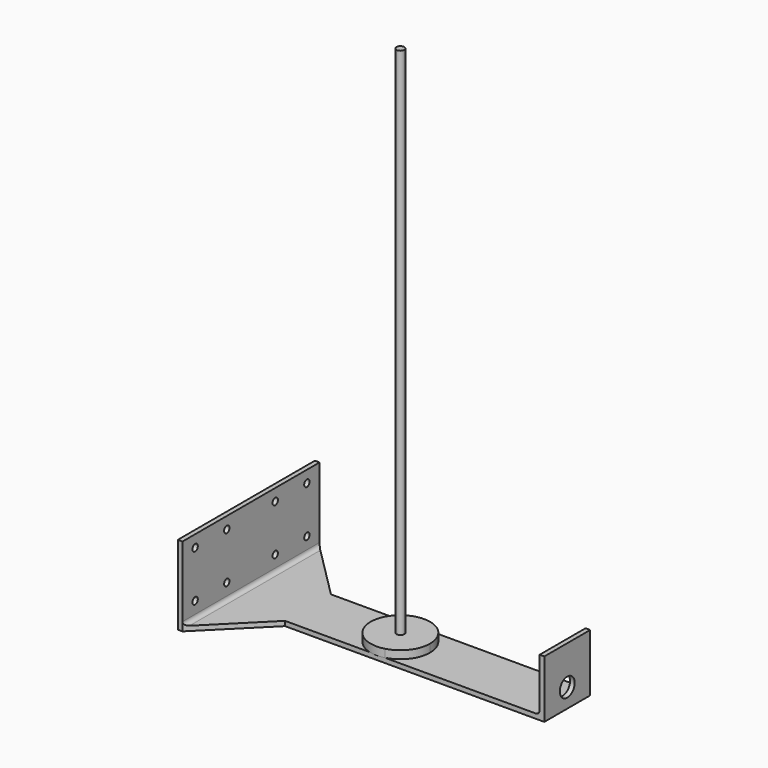
from build123d import *

# Parameters (mm, degrees)
F0_W      = 2.999994
F0_H      = 110.000034
F0_H_2    = 36.83
F1_DEPTH  = 2.999994
F2_DEPTH  = 50.8
F3_DEPTH  = 36.999926
F4_R      = 2.1499957
F5_DEPTH  = 49.276
F6_R      = 5.969
F7_DEPTH  = 38.1
F8_R      = 2.54
F10_DEPTH = 5.08
F11_R     = 2.54
F12_DEPTH = 330.2
F13_R     = 2.54


with BuildPart() as f1:
    # F0 (on Top) → F1 (new body)
    with BuildSketch(Plane.XY):
        Rectangle(F0_W, F0_H)
        Polygon((38.085014, 18.415), (1.499997, 55.000017), (1.499997, -55.000017), (38.085014, -18.415), (201.500105, -18.415), (201.500105, 18.415), align=None)
        with Locations((203.000102, 0)):
            Rectangle(F0_W, F0_H_2)
    extrude(amount=F1_DEPTH)

    # F0 (on Top) → F2 (join)
    with BuildSketch(Plane.XY):
        Rectangle(F0_W, F0_H)
    extrude(amount=F2_DEPTH)

    # F0 (on Top) → F3 (join)
    with BuildSketch(Plane.XY):
        with Locations((203.000102, 0)):
            Rectangle(F0_W, F0_H_2)
    extrude(amount=F3_DEPTH)

    # F4 (on face) → F5 (cut)
    with BuildSketch(Plane.YZ.offset(1.499997)):
        with Locations((-44.840017, 43.18)):
            Circle(F4_R)
        with Locations((-44.840017, 13.18006)):
            Circle(F4_R)
        with Locations((-19.440017, 43.18)):
            Circle(F4_R)
        with Locations((-19.440017, 13.18006)):
            Circle(F4_R)
        with Locations((44.840017, 43.18)):
            Circle(F4_R)
        with Locations((19.440017, 43.18)):
            Circle(F4_R)
        with Locations((19.440017, 13.18006)):
            Circle(F4_R)
        with Locations((44.840017, 13.18006)):
            Circle(F4_R)
    extrude(amount=-F5_DEPTH, mode=Mode.SUBTRACT)

    # F6 (on face) → F7 (cut)
    with BuildSketch(Plane.YZ.offset(204.500099)):
        with Locations((0, 12.192)):
            Circle(F6_R)
    extrude(amount=-F7_DEPTH, mode=Mode.SUBTRACT)

    # F8
    f8_edges = [f1.edges().sort_by_distance(p)[0] for p in [
        (201.500105, 0, 2.999994),
    ]]
    fillet(f8_edges, radius=F8_R)

    # F9 (on face) → F10 (join)
    with BuildSketch(Plane.XY.offset(2.999994)):
        with BuildLine():
            ThreePointArc((92.4825774501, -18.415), (97.360105, -19.05), (102.2376325499, -18.415))
            Line((102.2376325499, -18.415), (92.4825774501, -18.415))
        make_face()
        with BuildLine():
            ThreePointArc((102.2376325499, -18.415), (112.4567834397, -11.6186401996), (116.410105, 0))
            ThreePointArc((116.410105, 0), (112.4567834397, 11.6186401996), (102.2376325499, 18.415))
            Line((102.2376325499, 18.415), (92.4825774501, 18.415))
            ThreePointArc((92.4825774501, 18.415), (78.310105, 0), (92.4825774501, -18.415))
            Line((92.4825774501, -18.415), (102.2376325499, -18.415))
        make_face()
        with BuildLine():
            Line((92.4825774501, 18.415), (102.2376325499, 18.415))
            ThreePointArc((102.2376325499, 18.415), (97.360105, 19.05), (92.4825774501, 18.415))
        make_face()
    extrude(amount=F10_DEPTH)

    # F11 (on face) → F12 (join)
    with BuildSketch(Plane.XY.offset(8.079994)):
        with Locations((97.360105, 0)):
            Circle(F11_R)
    extrude(amount=F12_DEPTH)

    # F13
    f13_edges = [f1.edges().sort_by_distance(p)[0] for p in [
        (1.499997, 0, 2.999994),
    ]]
    fillet(f13_edges, radius=F13_R)


solid = f1.part
